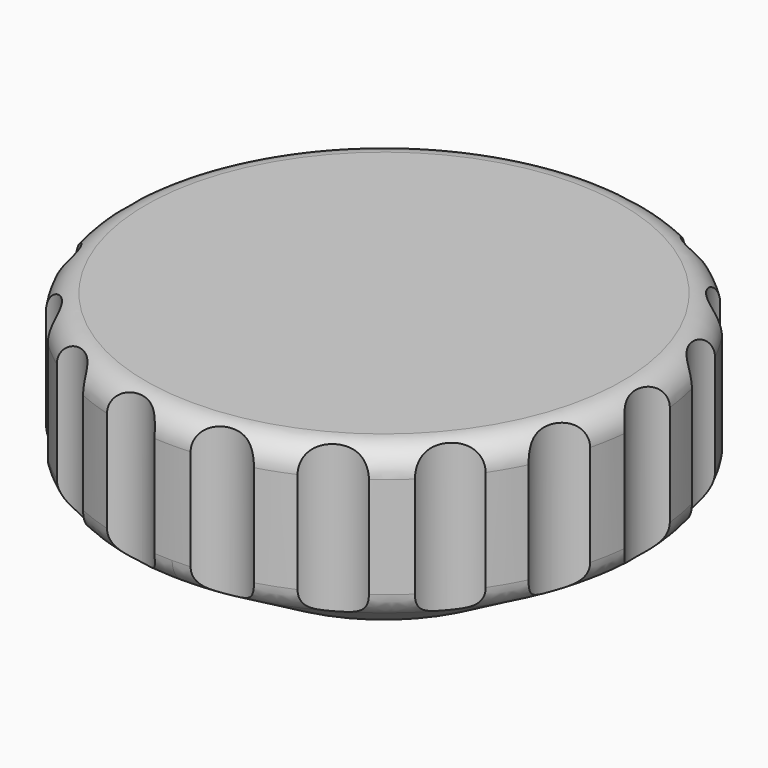
from build123d import *

# Parameters (mm, degrees)
F2_R     = 1
F4_DEPTH = 4
F5_R     = 1.5
F6_DEPTH = 8.0010001


with BuildPart() as f1:
    # F0 (on Right) → F1 (revolve)
    with BuildSketch(Plane.YZ):
        Polygon((0, 4), (0, 8), (-10, 8), (-10, 2.5980762114), (-5.5, 0), (-3.5, 0), (-3.5, 4), align=None)
    revolve(axis=Axis((0, 0, 3.5727035735), (0, 0, 1)))

    # F2
    f2_edges = [f1.edges().sort_by_distance(p)[0] for p in [
        (0, 10, 8),
        (0, 10, 2.598076),
    ]]
    fillet(f2_edges, radius=F2_R)

    # F3 (on face) → F4 (cut, through all)
    with BuildSketch(Plane(origin=(0, 0, 0), x_dir=(1, 0, 0), z_dir=(0, 0, -1))):
        with BuildLine():
            ThreePointArc((-3.4818181818, -0.3562894171), (-3.5, 0), (-3.4818181818, 0.3562894171))
            ThreePointArc((-3.4818181818, 0.3562894171), (-3.7, 0), (-3.4818181818, -0.3562894171))
        make_face()
        with BuildLine():
            ThreePointArc((-2.6074284155, 2.3348055718), (-2.8315594803, 2.057248383), (-3.0262717454, 1.7583171851))
            ThreePointArc((-3.0262717454, 1.7583171851), (-2.5764990859, 1.5507142988), (-2.2697560814, 1.9396913326))
            ThreePointArc((-2.2697560814, 1.9396913326), (-2.3656746233, 2.1995652766), (-2.6074284155, 2.3348055718))
        make_face()
        with BuildLine():
            ThreePointArc((-2.6074284155, 2.3348055718), (-2.9933628792, 2.1748054335), (-3.0262717454, 1.7583171851))
            ThreePointArc((-3.0262717454, 1.7583171851), (-2.8315594803, 2.057248383), (-2.6074284155, 2.3348055718))
        make_face()
        with BuildLine():
            ThreePointArc((-2.6074284155, -2.3348055718), (-2.8315594803, -2.057248383), (-3.0262717454, -1.7583171851))
            ThreePointArc((-3.0262717454, -1.7583171851), (-2.9933628792, -2.1748054335), (-2.6074284155, -2.3348055718))
        make_face()
        with BuildLine():
            ThreePointArc((-0.7370896177, 3.4215053552), (-1.0815594803, 3.328697807), (-1.4147923614, 3.2013063856))
            ThreePointArc((-1.4147923614, 3.2013063856), (-1.051263922, 2.7397293647), (-0.6197560814, 3.1384865038))
            ThreePointArc((-0.6197560814, 3.1384865038), (-0.6502519641, 3.2916749735), (-0.7370896177, 3.4215053552))
        make_face()
        with BuildLine():
            ThreePointArc((-0.7370896177, 3.4215053552), (-1.1433628792, 3.5189091103), (-1.4147923614, 3.2013063856))
            ThreePointArc((-1.4147923614, 3.2013063856), (-1.0815594803, 3.328697807), (-0.7370896177, 3.4215053552))
        make_face()
        with BuildLine():
            ThreePointArc((-0.7370896177, -3.4215053552), (-1.0815594803, -3.328697807), (-1.4147923614, -3.2013063856))
            ThreePointArc((-1.4147923614, -3.2013063856), (-1.1433628792, -3.5189091103), (-0.7370896177, -3.4215053552))
        make_face()
        with BuildLine():
            ThreePointArc((1.4147923614, 3.2013063856), (1.0815594803, 3.328697807), (0.7370896177, 3.4215053552))
            ThreePointArc((0.7370896177, 3.4215053552), (0.8665676118, 2.7689823864), (1.4197560814, 3.1384865038))
            ThreePointArc((1.4197560814, 3.1384865038), (1.4185132205, 3.1699943443), (1.4147923614, 3.2013063856))
        make_face()
        with BuildLine():
            ThreePointArc((1.4147923614, 3.2013063856), (1.1433628792, 3.5189091103), (0.7370896177, 3.4215053552))
            ThreePointArc((0.7370896177, 3.4215053552), (1.0815594803, 3.328697807), (1.4147923614, 3.2013063856))
        make_face()
        with BuildLine():
            ThreePointArc((1.4147923614, -3.2013063856), (1.0815594803, -3.328697807), (0.7370896177, -3.4215053552))
            ThreePointArc((0.7370896177, -3.4215053552), (1.1433628792, -3.5189091103), (1.4147923614, -3.2013063856))
        make_face()
        with BuildLine():
            ThreePointArc((3.0262717454, 1.7583171851), (2.8315594803, 2.057248383), (2.6074284155, 2.3348055718))
            ThreePointArc((2.6074284155, 2.3348055718), (2.3461492837, 1.7045772316), (3.0262717454, 1.7583171851))
        make_face()
        with BuildLine():
            ThreePointArc((3.0697560814, 1.9396913326), (2.9296300255, 2.2437727907), (2.6074284155, 2.3348055718))
            ThreePointArc((2.6074284155, 2.3348055718), (2.8315594803, 2.057248383), (3.0262717454, 1.7583171851))
            ThreePointArc((3.0262717454, 1.7583171851), (3.0587331152, 1.846434337), (3.0697560814, 1.9396913326))
        make_face()
        with BuildLine():
            ThreePointArc((3.0262717454, -1.7583171851), (2.8315594803, -2.057248383), (2.6074284155, -2.3348055718))
            ThreePointArc((2.6074284155, -2.3348055718), (2.9296300255, -2.2437727907), (3.0697560814, -1.9396913326))
            ThreePointArc((3.0697560814, -1.9396913326), (3.0587331152, -1.846434337), (3.0262717454, -1.7583171851))
        make_face()
        with BuildLine():
            ThreePointArc((3.7, 0), (3.6411211462, 0.2088931871), (3.4818181818, 0.3562894171))
            ThreePointArc((3.4818181818, 0.3562894171), (3.49545159, 0.178376517), (3.5, 0))
            ThreePointArc((3.5, 0), (3.49545159, -0.178376517), (3.4818181818, -0.3562894171))
            ThreePointArc((3.4818181818, -0.3562894171), (3.6411211462, -0.2088931871), (3.7, 0))
        make_face()
    extrude(amount=-F4_DEPTH, mode=Mode.SUBTRACT)

    # F5 (on face) → F6 (cut, through all)
    with BuildSketch(Plane.XY.offset(8)):
        with Locations((11, 0)):
            Circle(F5_R)
        with Locations((10.3366188286, 3.7622215766)):
            Circle(F5_R)
        with Locations((8.4264888743, 7.0706637066)):
            Circle(F5_R)
        with Locations((5.5, 9.5262794416)):
            Circle(F5_R)
        with Locations((1.9101299543, 10.8328852831)):
            Circle(F5_R)
        with Locations((-1.9101299543, 10.8328852831)):
            Circle(F5_R)
        with Locations((-5.5, 9.5262794416)):
            Circle(F5_R)
        with Locations((-8.4264888743, 7.0706637066)):
            Circle(F5_R)
        with Locations((-10.3366188286, 3.7622215766)):
            Circle(F5_R)
        with Locations((-11, 0)):
            Circle(F5_R)
        with Locations((-10.3366188286, -3.7622215766)):
            Circle(F5_R)
        with Locations((-8.4264888743, -7.0706637066)):
            Circle(F5_R)
        with Locations((-5.5, -9.5262794416)):
            Circle(F5_R)
        with Locations((-1.9101299543, -10.8328852831)):
            Circle(F5_R)
        with Locations((1.9101299543, -10.8328852831)):
            Circle(F5_R)
        with Locations((5.5, -9.5262794416)):
            Circle(F5_R)
        with Locations((8.4264888743, -7.0706637066)):
            Circle(F5_R)
        with Locations((10.3366188286, -3.7622215766)):
            Circle(F5_R)
    extrude(amount=-F6_DEPTH, mode=Mode.SUBTRACT)


solid = f1.part
